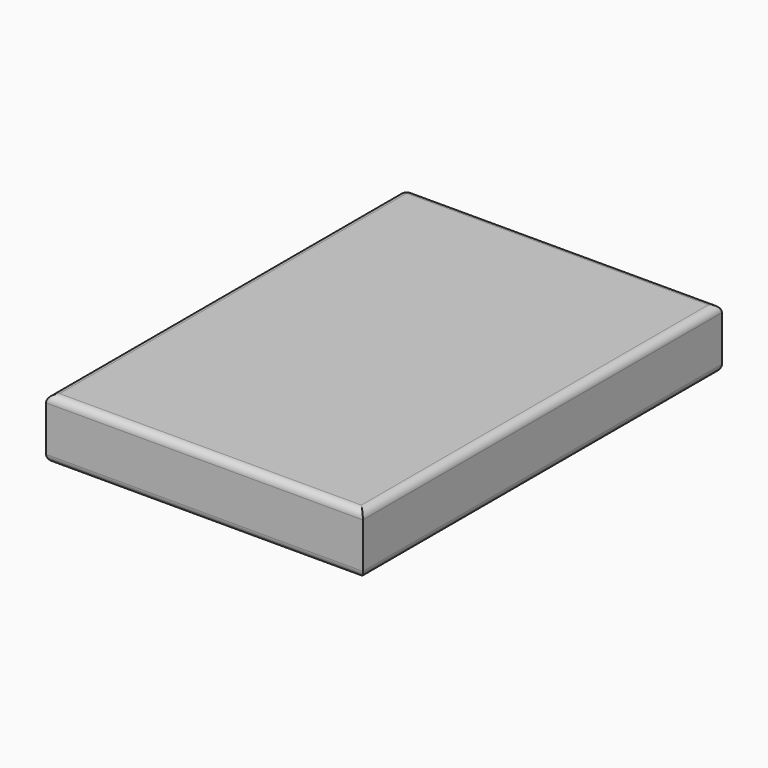
from build123d import *

# Parameters (mm, degrees)
F0_W         = 84
F0_H         = 119
F1_DEPTH     = 16
F2_W         = 23.2555542788
F2_H         = 5.3250671498
F3_DEPTH     = 13
F4_R         = 2
F5_T1_DEPTH  = 122
F5_T3_DEPTH  = 94
F5_T5_DEPTH  = 129
F5_T7_DEPTH  = 41.8466055248
F5_T9_DEPTH  = 12
F5_S13_W     = 2
F5_S13_H     = 2
F5_T14_DEPTH = 2
F5_T18_ANGLE = 90
F7_DEPTH     = 2
F8_T1_DEPTH  = 90.4739352316
F8_T3_DEPTH  = 90.5


# Not quite as in the source:
# - a fillet or chamfer that OpenCascade refuses, or shapes differently, is made with other operations: its cross-section is extruded or revolved along the edge and cut away or added


with BuildPart() as f1:
    # F0 (on Top) → F1 (new body)
    with BuildSketch(Plane.XY):
        with Locations((19.1573249176, -12.7916212418)):
            Rectangle(F0_W, F0_H)
    extrude(amount=F1_DEPTH)

    # F2 (on Top) → F3 (cut)
    with BuildSketch(Plane.XY):
        Polygon((6.055165114, 44.0079532564), (-21.2180707604, 44.0079532564), (-21.2180707604, -69.7137644664), (59.2819292396, -69.7137644664), (59.2819292396, 44.0079532564), (29.3107193928, 44.0079532564), align=None)
        with Locations((17.6829422534, 46.6704868313)):
            Rectangle(F2_W, F2_H)
    extrude(amount=F3_DEPTH, mode=Mode.SUBTRACT)

    # F4
    f4_edges = [f1.edges().sort_by_distance(p)[0] for p in [
        (61.157325, -12.791621, 16),
        (19.157325, -72.291621, 16),
        (-22.842675, -12.791621, 16),
        (19.157325, 46.708379, 16),
        (-8.393755, 46.708379, 0),
    ]]
    fillet(f4_edges, radius=F4_R)

    # F5: fillet of radius 2 on 4 edges, made by hand

    # F5_s2 → F5_t1 (cut)
    with BuildSketch(Plane.XZ.offset(-44.7083787582)):
        with BuildLine():
            ThreePointArc((-22.8426750824, 2), (-22.2568886448, 0.5857864376), (-20.8426750824, 0))
            Line((-20.8426750824, 0), (-22.8426750824, 0))
            Line((-22.8426750824, 0), (-22.8426750824, 2))
        make_face()
    extrude(amount=F5_T1_DEPTH, mode=Mode.SUBTRACT)

    # F5_s4 → F5_t3 (cut)
    with BuildSketch(Plane.YZ.offset(-27.8426750824)):
        with BuildLine():
            ThreePointArc((-70.2916212418, 0), (-71.7058348042, 0.5857864376), (-72.2916212418, 2))
            Line((-72.2916212418, 2), (-72.2916212418, 0))
            Line((-72.2916212418, 0), (-70.2916212418, 0))
        make_face()
    extrude(amount=F5_T3_DEPTH, mode=Mode.SUBTRACT)

    # F5_s6 → F5_t5 (cut)
    with BuildSketch(Plane.XZ.offset(-51.7083787582)):
        with BuildLine():
            ThreePointArc((59.1573249176, 0), (60.57153848, 0.5857864376), (61.1573249176, 2))
            Line((61.1573249176, 2), (61.1573249176, 0))
            Line((61.1573249176, 0), (59.1573249176, 0))
        make_face()
    extrude(amount=F5_T5_DEPTH, mode=Mode.SUBTRACT)

    # F5_s8 → F5_t7 (cut)
    with BuildSketch(Plane.YZ.offset(24.3107193928)):
        with BuildLine():
            ThreePointArc((46.7083787582, 2), (46.1225923205, 0.5857864376), (44.7083787582, 0))
            Line((44.7083787582, 0), (46.7083787582, 0))
            Line((46.7083787582, 0), (46.7083787582, 2))
        make_face()
    extrude(amount=F5_T7_DEPTH, mode=Mode.SUBTRACT)

    # F5_s10 → F5_t9 (cut)
    with BuildSketch(Plane.XY.offset(2)):
        with BuildLine():
            ThreePointArc((-20.8426750824, 46.7083787582), (-22.2568886448, 46.1225923205), (-22.8426750824, 44.7083787582))
            Line((-22.8426750824, 44.7083787582), (-22.8426750824, 46.7083787582))
            Line((-22.8426750824, 46.7083787582), (-20.8426750824, 46.7083787582))
        make_face()
    extrude(amount=F5_T9_DEPTH, mode=Mode.SUBTRACT)


with BuildPart() as f5_tool12:
    # F5_s13 → F5_t14 (new body)
    with BuildSketch(Plane.XZ.offset(-44.7083787582)):
        with Locations((-21.8426750824, 15)):
            Rectangle(F5_S13_W, F5_S13_H)
    extrude(amount=-F5_T14_DEPTH)

    # F5_s15 → F5_t16 (revolve, cut)
    with BuildSketch(Plane(origin=(-20.8426750824, 44.7083787582, 14), x_dir=(0.7071067812, 0, -0.7071067812), z_dir=(0.7071067812, 0, 0.7071067812))):
        with BuildLine():
            ThreePointArc((0, -2), (2, 0), (0, 2))
            Line((0, 2), (0, -2))
        make_face()
    revolve(axis=Axis((-20.8426750824, 44.7083787582, 14), (0, 1, 0)), mode=Mode.SUBTRACT)


with BuildPart() as f1_1:
    add(f1.part)

    # F5_t11: cut F5_tool12
    add(f5_tool12.part, mode=Mode.SUBTRACT)

    # F5_s17 → F5_t18 (revolve, cut)
    with BuildSketch(Plane.XY.offset(2)):
        with BuildLine():
            ThreePointArc((-20.8426750824, 46.7083787582), (-22.2568886448, 46.1225923205), (-22.8426750824, 44.7083787582))
            Line((-22.8426750824, 44.7083787582), (-22.8426750824, 46.7083787582))
            Line((-22.8426750824, 46.7083787582), (-20.8426750824, 46.7083787582))
        make_face()
    revolve(axis=Axis((-22.8426750824, 44.7083787582, 2), (-1, 0, 0)), revolution_arc=F5_T18_ANGLE, mode=Mode.SUBTRACT)


with BuildPart() as f7:
    # F6 (on Top) → F7 (new body)
    with BuildSketch(Plane.XY):
        Polygon((59.5953304619, -7.7894940041), (-20.9046695381, -7.7894940041), (-20.9046695381, -17.5308659673), (59.5692656934, -17.5308659673), align=None)
    extrude(amount=F7_DEPTH)

    # F8: fillet of radius 2 on 4 edges, made by hand

    # F8_s2 → F8_t1 (cut)
    with BuildSketch(Plane.YZ.offset(-25.9046695381)):
        with BuildLine():
            ThreePointArc((-17.5308659673, 2), (-16.9450795296, 0.5857864376), (-15.5308659673, 0))
            Line((-15.5308659673, 0), (-17.5308659673, 0))
            Line((-17.5308659673, 0), (-17.5308659673, 2))
        make_face()
        with BuildLine():
            ThreePointArc((-17.5308659673, 0), (-16.9450795296, 1.4142135624), (-15.5308659673, 2))
            Line((-15.5308659673, 2), (-17.5308659673, 2))
            Line((-17.5308659673, 2), (-17.5308659673, 0))
        make_face()
    extrude(amount=F8_T1_DEPTH, mode=Mode.SUBTRACT)

    # F8_s4 → F8_t3 (cut)
    with BuildSketch(Plane.YZ.offset(-25.9046695381)):
        with BuildLine():
            ThreePointArc((-7.7894940041, 2), (-8.3752804417, 0.5857864376), (-9.7894940041, 0))
            Line((-9.7894940041, 0), (-7.7894940041, 0))
            Line((-7.7894940041, 0), (-7.7894940041, 2))
        make_face()
        with BuildLine():
            ThreePointArc((-7.7894940041, 0), (-8.3752804417, 1.4142135624), (-9.7894940041, 2))
            Line((-9.7894940041, 2), (-7.7894940041, 2))
            Line((-7.7894940041, 2), (-7.7894940041, 0))
        make_face()
    extrude(amount=F8_T3_DEPTH, mode=Mode.SUBTRACT)


solid = Compound([f1_1.part, f7.part])
